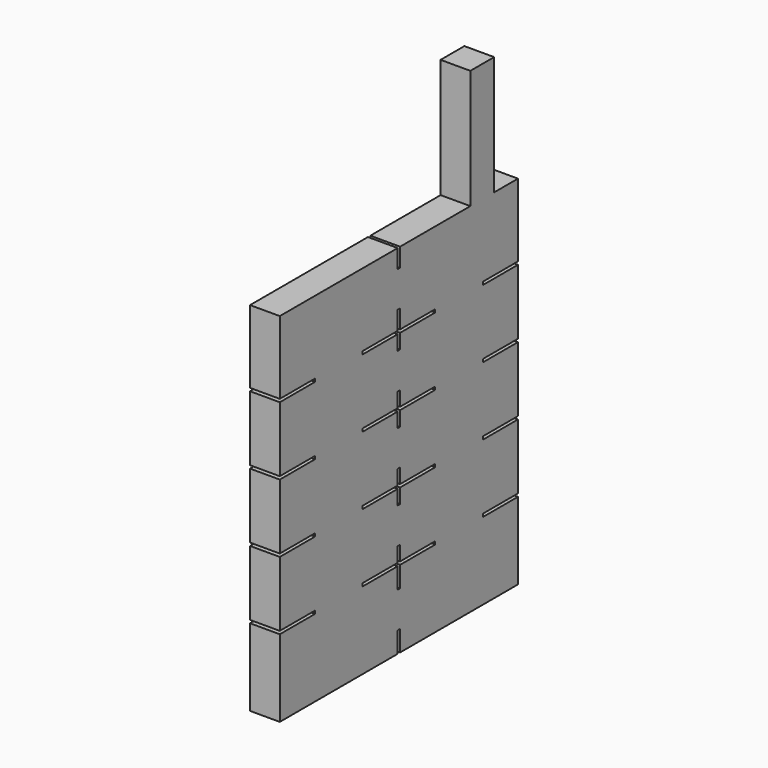
from build123d import *

# Parameters (mm, degrees)
F1_DEPTH = 5


# Not quite as in the source:
# - a feature names something its author has since deleted; it is built from what else it names


with BuildPart() as f1:
    # F0 (on Right) → F1 (new body)
    with BuildSketch(Plane.YZ):
        Polygon((11.5, 0), (0, 0), (0, -12.238), (7.3750000447, -12.238), (7.3750000447, -12.738), (0, -12.738), (0, -23.672), (7.3750000447, -23.672), (7.3750000447, -24.172), (0, -24.172), (0, -35.106), (7.3750000447, -35.106), (7.3750000447, -35.606), (0, -35.606), (0, -46.54), (7.3750000447, -46.54), (7.3750000447, -47.04), (0, -47.04), (0, -60), (24.75, -60), (24.75, -56.52), (25.25, -56.52), (25.25, -60), (50, -60), (50, -47.04), (42.6249988377, -47.04), (42.6249988377, -46.54), (50, -46.54), (50, -35.606), (42.6249988377, -35.606), (42.6249988377, -35.106), (50, -35.106), (50, -24.172), (42.6249988377, -24.172), (42.6249988377, -23.672), (50, -23.672), (50, -12.738), (42.6249988377, -12.738), (42.6249988377, -12.238), (50, -12.238), (50, 0), (45, 0), (45, 15), (45, 19.999999553), (40, 19.999999553), (40, 15), (40, 0), (37.625, 0), (35.125, 0), (25.25, 0), (25.25, -1.304), (25.25, -3.119), (24.75, -3.119), (24.75, 0), (14.875, 0), (12.375, 0), align=None)
        Polygon((25.25, -44.073), (25.25, -46.54), (32.625, -46.54), (32.625, -47.04), (25.25, -47.04), (25.25, -50.52), (24.75, -50.52), (24.75, -47.04), (17.375, -47.04), (17.375, -46.54), (24.75, -46.54), (24.75, -44.073), align=None, mode=Mode.SUBTRACT)
        Polygon((25.25, -32.639), (25.25, -35.106), (32.625, -35.106), (32.625, -35.606), (25.25, -35.606), (25.25, -38.073), (24.75, -38.073), (24.75, -35.606), (17.375, -35.606), (17.375, -35.106), (24.75, -35.106), (24.75, -32.639), align=None, mode=Mode.SUBTRACT)
        Polygon((25.25, -21.205), (25.25, -23.672), (32.625, -23.672), (32.625, -24.172), (25.25, -24.172), (25.25, -26.639), (24.75, -26.639), (24.75, -24.172), (17.375, -24.172), (17.375, -23.672), (24.75, -23.672), (24.75, -21.205), align=None, mode=Mode.SUBTRACT)
        Polygon((25.25, -9.119), (25.25, -12.238), (32.625, -12.238), (32.625, -12.738), (25.25, -12.738), (25.25, -15.205), (24.75, -15.205), (24.75, -12.738), (17.375, -12.738), (17.375, -12.238), (24.75, -12.238), (24.75, -9.119), align=None, mode=Mode.SUBTRACT)
    extrude(amount=F1_DEPTH)


solid = f1.part
